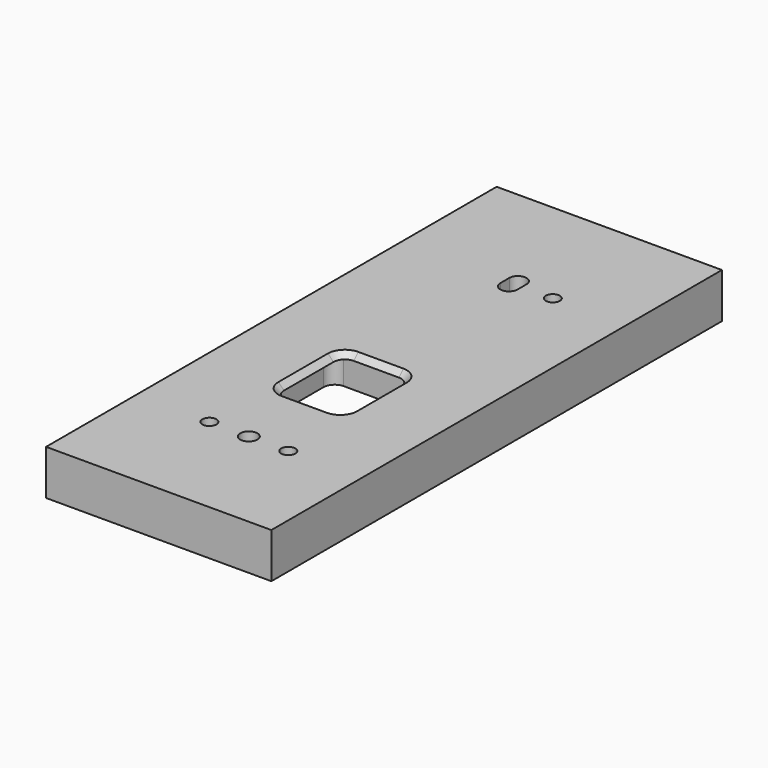
from build123d import *

# Parameters (mm, degrees)
F0_W     = 40
F0_H     = 100
F0_R     = 1.25
F0_R_2   = 1.525
F1_DEPTH = 8
F2_DEPTH = 7
F3_DEPTH = 5
F4_SIZE  = 0.99999


# Not quite as in the source:
# - a fillet or chamfer is up to 0.001 mm smaller than in the source, because OpenCascade refuses the exact size


with BuildPart() as f1:
    # F0 (on Top) → F1 (new body)
    with BuildSketch(Plane.XY):
        with Locations((0, 30)):
            Rectangle(F0_W, F0_H)
        with Locations((-7, 0)):
            Circle(F0_R, mode=Mode.SUBTRACT)
        Circle(F0_R_2, mode=Mode.SUBTRACT)
        with Locations((7, 0)):
            Circle(F0_R, mode=Mode.SUBTRACT)
        with BuildLine():
            ThreePointArc((-10.75, 30), (-10.1642135624, 31.4142135624), (-8.75, 32))
            Line((-8.75, 32), (8.75, 32))
            ThreePointArc((8.75, 32), (10.1642135624, 31.4142135624), (10.75, 30))
            Line((10.75, 30), (10.75, 11.6))
            Line((10.75, 11.6), (10.75, 5.5))
            ThreePointArc((10.75, 5.5), (8.75, 3.5), (6.75, 5.5))
            Line((6.75, 5.5), (-6.75, 5.5))
            ThreePointArc((-6.75, 5.5), (-8.75, 3.5), (-10.75, 5.5))
            Line((-10.75, 5.5), (-10.75, 11.6))
            Line((-10.75, 11.6), (-10.75, 30))
        make_face(mode=Mode.SUBTRACT)
        with BuildLine():
            Line((-1.53, 57.72), (-1.53, 59.72))
            ThreePointArc((-1.53, 59.72), (0, 61.25), (1.53, 59.72))
            Line((1.53, 59.72), (1.53, 57.72))
            ThreePointArc((1.53, 57.72), (0, 56.19), (-1.53, 57.72))
        make_face(mode=Mode.SUBTRACT)
        with Locations((7, 58.72)):
            Circle(F0_R, mode=Mode.SUBTRACT)
        with BuildLine():
            Line((8.75, 32), (-8.75, 32))
            ThreePointArc((-8.75, 32), (-10.1642135624, 31.4142135624), (-10.75, 30))
            Line((-10.75, 30), (-10.75, 11.6))
            ThreePointArc((-10.75, 11.6), (-10.1642135624, 10.1857864376), (-8.75, 9.6))
            Line((-8.75, 9.6), (8.75, 9.6))
            ThreePointArc((8.75, 9.6), (10.1642135624, 10.1857864376), (10.75, 11.6))
            Line((10.75, 11.6), (10.75, 30))
            ThreePointArc((10.75, 30), (10.1642135624, 31.4142135624), (8.75, 32))
        make_face()
        with BuildLine():
            ThreePointArc((-6, 26.3), (-5.4142135624, 27.7142135624), (-4, 28.3))
            Line((-4, 28.3), (4, 28.3))
            ThreePointArc((4, 28.3), (5.4142135624, 27.7142135624), (6, 26.3))
            Line((6, 26.3), (6, 15.3))
            ThreePointArc((6, 15.3), (5.4142135624, 13.8857864376), (4, 13.3))
            Line((4, 13.3), (-4, 13.3))
            ThreePointArc((-4, 13.3), (-5.4142135624, 13.8857864376), (-6, 15.3))
            Line((-6, 15.3), (-6, 26.3))
        make_face(mode=Mode.SUBTRACT)
        with BuildLine():
            ThreePointArc((-8.75, 9.6), (-10.1642135624, 10.1857864376), (-10.75, 11.6))
            Line((-10.75, 11.6), (-10.75, 5.5))
            ThreePointArc((-10.75, 5.5), (-8.75, 3.5), (-6.75, 5.5))
            Line((-6.75, 5.5), (6.75, 5.5))
            ThreePointArc((6.75, 5.5), (8.75, 3.5), (10.75, 5.5))
            Line((10.75, 5.5), (10.75, 11.6))
            ThreePointArc((10.75, 11.6), (10.1642135624, 10.1857864376), (8.75, 9.6))
            Line((8.75, 9.6), (-8.75, 9.6))
        make_face()
    extrude(amount=F1_DEPTH)

    # F0 (on Top) → F2 (cut)
    with BuildSketch(Plane.XY):
        with BuildLine():
            Line((8.75, 32), (-8.75, 32))
            ThreePointArc((-8.75, 32), (-10.1642135624, 31.4142135624), (-10.75, 30))
            Line((-10.75, 30), (-10.75, 11.6))
            ThreePointArc((-10.75, 11.6), (-10.1642135624, 10.1857864376), (-8.75, 9.6))
            Line((-8.75, 9.6), (8.75, 9.6))
            ThreePointArc((8.75, 9.6), (10.1642135624, 10.1857864376), (10.75, 11.6))
            Line((10.75, 11.6), (10.75, 30))
            ThreePointArc((10.75, 30), (10.1642135624, 31.4142135624), (8.75, 32))
        make_face()
        with BuildLine():
            ThreePointArc((-6, 26.3), (-5.4142135624, 27.7142135624), (-4, 28.3))
            Line((-4, 28.3), (4, 28.3))
            ThreePointArc((4, 28.3), (5.4142135624, 27.7142135624), (6, 26.3))
            Line((6, 26.3), (6, 15.3))
            ThreePointArc((6, 15.3), (5.4142135624, 13.8857864376), (4, 13.3))
            Line((4, 13.3), (-4, 13.3))
            ThreePointArc((-4, 13.3), (-5.4142135624, 13.8857864376), (-6, 15.3))
            Line((-6, 15.3), (-6, 26.3))
        make_face(mode=Mode.SUBTRACT)
    extrude(amount=F2_DEPTH, mode=Mode.SUBTRACT)

    # F0 (on Top) → F3 (cut)
    with BuildSketch(Plane.XY):
        with BuildLine():
            ThreePointArc((-8.75, 9.6), (-10.1642135624, 10.1857864376), (-10.75, 11.6))
            Line((-10.75, 11.6), (-10.75, 5.5))
            ThreePointArc((-10.75, 5.5), (-8.75, 3.5), (-6.75, 5.5))
            Line((-6.75, 5.5), (6.75, 5.5))
            ThreePointArc((6.75, 5.5), (8.75, 3.5), (10.75, 5.5))
            Line((10.75, 5.5), (10.75, 11.6))
            ThreePointArc((10.75, 11.6), (10.1642135624, 10.1857864376), (8.75, 9.6))
            Line((8.75, 9.6), (-8.75, 9.6))
        make_face()
    extrude(amount=F3_DEPTH, mode=Mode.SUBTRACT)

    # F4 (size 1 in the source; OpenCascade refuses exactly that, so slightly less here)
    f4_edges = [f1.edges().sort_by_distance(p)[0] for p in [
        (6, 20.8, 8),
        (5.414214, 13.885786, 8),
        (0, 13.3, 8),
        (-5.414214, 13.885786, 8),
        (-6, 20.8, 8),
        (-5.414214, 27.714214, 8),
        (0, 28.3, 8),
        (5.414214, 27.714214, 8),
    ]]
    chamfer(f4_edges, length=F4_SIZE)


solid = f1.part
